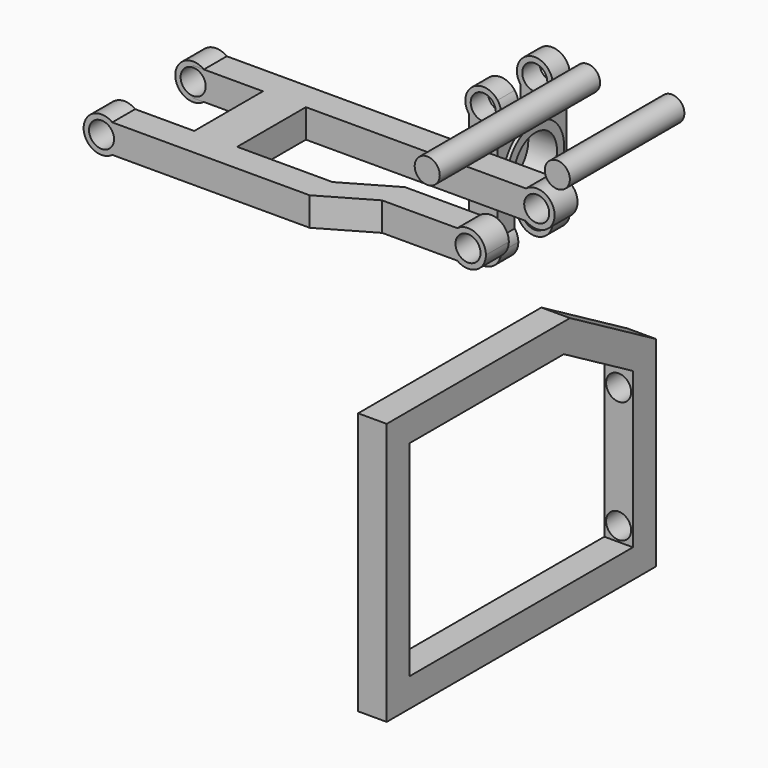
from build123d import *

# Parameters (mm, degrees)
F0_W      = 304.8
F0_H      = 25.4
F1_DEPTH  = 25.4
F4_DEPTH  = 25.4
F5_DEPTH  = 25.4
F7_DEPTH  = 25.4
F8_R      = 11.1125
F9_DEPTH  = 127.001
F10_R     = 11.1125
F11_DEPTH = 101.601
F12_R     = 11.1125
F13_DEPTH = 127.001
F14_W     = 38.1
F14_H     = 86.0915481232
F15_DEPTH = 25.4
F16_DEPTH = 25.4
F19_DEPTH = 12.7
F20_DEPTH = 12.7
F18_R     = 6.35
F21_DEPTH = 15.875
F23_DEPTH = 19.05
F24_DEPTH = 211.7314750923
F26_DEPTH = 19.05
F27_R     = 23.8125
F28_DEPTH = 25.4
F29_R     = 11.1125
F30_DEPTH = 127
F33_DEPTH = 25.4
F34_R     = 11.1125
F35_DEPTH = 25.4
F31_R     = 11.1125
F36_DEPTH = 177.8


# Not quite as in the source:
# - a pattern or mirror of a feature is missing from the dataset's text; its kind, count and spacing are read off the source's solid


with BuildPart() as f1:
    # F0 (on Top) → F1 (new body)
    with BuildSketch(Plane.XY):
        with Locations((-77.8089873464, -4.2339627839)):
            Rectangle(F0_W, F0_H)
    extrude(amount=F1_DEPTH)



with BuildPart() as f1b:
    # F0 (on Top) → F1, piece 2 (new body)
    with BuildSketch(Plane.XY):
        Polygon((-230.2089873464, -93.1339627839), (-230.2089873464, -118.5339627839), (-45.6030778587, -118.5339627839), (-1.6089873464, -93.1339627839), (74.5910126536, -93.1339627839), (74.5910126536, -67.7339627839), (-1.6089873464, -67.7339627839), (-45.6030778587, -93.1339627839), align=None)
    extrude(amount=F1_DEPTH)

    # F2 (on face) → F4 (join)
    with BuildSketch(Plane.XZ.offset(118.5339627839)):
        with BuildLine():
            Line((-230.2089873464, 25.4), (-220.6839873464, 25.4))
            ThreePointArc((-220.6839873464, 25.4), (-246.0839873464, 12.7), (-220.6839873464, 0))
            Line((-220.6839873464, 0), (-230.2089873464, 0))
            Line((-230.2089873464, 0), (-230.2089873464, 25.4))
        make_face()
    f4 = extrude(amount=-F4_DEPTH)

    # F4_copies: F4 across plane
    add(f4.mirror(Plane.ZX.offset(-55.033963)))

    # F3 (on face) → F5 (join)
    with BuildSketch(Plane.XZ.offset(93.1339627839)):
        with BuildLine():
            ThreePointArc((65.0660126536, 0), (81.6905284821, -1.4990316571), (90.4660126536, 12.7))
            ThreePointArc((90.4660126536, 12.7), (81.6905284821, 26.8990316571), (65.0660126536, 25.4))
            Line((65.0660126536, 25.4), (74.5910126536, 25.4))
            Line((74.5910126536, 25.4), (74.5910126536, 0))
            Line((74.5910126536, 0), (65.0660126536, 0))
        make_face()
        with BuildLine():
            Line((74.5910126536, 25.4), (65.0660126536, 25.4))
            ThreePointArc((65.0660126536, 25.4), (58.7160126536, 12.7), (65.0660126536, 0))
            Line((65.0660126536, 0), (74.5910126536, 0))
            Line((74.5910126536, 0), (74.5910126536, 25.4))
        make_face()
    extrude(amount=-F5_DEPTH)


with BuildPart() as f1_1:
    add(f1.part)

    add(f1b.part)  # F7 merges F1b
    # F6 (on face) → F7 (join)
    with BuildSketch(Plane(origin=(0, 8.4660372161, 0), x_dir=(-1, 0, 0), z_dir=(0, 1, 0))):
        with BuildLine():
            Line((-74.5910126536, 25.4), (-65.0660126536, 25.4))
            ThreePointArc((-65.0660126536, 25.4), (-90.4660126536, 12.7), (-65.0660126536, 0))
            Line((-65.0660126536, 0), (-74.5910126536, 0))
            Line((-74.5910126536, 0), (-74.5910126536, 25.4))
        make_face()
        with BuildLine():
            Line((230.2089873464, 25.4), (220.6839873464, 25.4))
            ThreePointArc((220.6839873464, 25.4), (214.3339873464, 12.7), (220.6839873464, 0))
            Line((220.6839873464, 0), (230.2089873464, 0))
            Line((230.2089873464, 0), (230.2089873464, 25.4))
        make_face()
    extrude(amount=-F7_DEPTH)

    # F8 (on face) → F9 (cut, through all)
    with BuildSketch(Plane.XZ.offset(118.5339627839)):
        with Locations((-230.2089873464, 12.7)):
            Circle(F8_R)
    extrude(amount=-F9_DEPTH, mode=Mode.SUBTRACT)

    # F10 (on face) → F11 (cut, through all)
    with BuildSketch(Plane.XZ.offset(93.1339627839)):
        with Locations((74.5910126536, 12.7)):
            Circle(F10_R)
    extrude(amount=-F11_DEPTH, mode=Mode.SUBTRACT)

    # F12 (on face) → F13 (cut, through all)
    with BuildSketch(Plane(origin=(0, 8.4660372161, 0), x_dir=(-1, 0, 0), z_dir=(0, 1, 0))):
        with Locations((-74.5910126536, 12.7)):
            Circle(F12_R)
        with BuildLine():
            ThreePointArc((230.2089873464, 1.5875), (238.0667114524, 4.8422758941), (241.3214873464, 12.7))
            ThreePointArc((241.3214873464, 12.7), (238.0667114524, 20.5577241059), (230.2089873464, 23.8125))
            ThreePointArc((230.2089873464, 23.8125), (222.3512632405, 20.5577241059), (219.0964873464, 12.7))
            ThreePointArc((219.0964873464, 12.7), (222.3512632405, 4.8422758941), (230.2089873464, 1.5875))
        make_face()
    extrude(amount=-F13_DEPTH, mode=Mode.SUBTRACT)

    # F14 (on face) → F15 (join)
    with BuildSketch(Plane.XY.offset(25.4)):
        with Locations((-149.2464873464, -59.9797368456)):
            Rectangle(F14_W, F14_H)
    extrude(amount=-F15_DEPTH)


with BuildPart() as f16:
    # F16 (new): a face of the model
    f16_faces = [f1_1.part.faces().sort_by_distance(p)[0] for p in [
        (-168.2964873464, -55.0339627839, 12.7),
    ]]
    extrude(f16_faces, amount=F16_DEPTH)


with BuildPart() as f19:
    # F18 (on Right) → F19 (new body, symmetric)
    with BuildSketch(Plane.YZ):
        with BuildLine():
            Line((36.0465123084, 63.5), (16.9965123084, 63.5))
            Line((16.9965123084, 63.5), (16.9965123084, -63.5))
            Line((16.9965123084, -63.5), (36.0465123084, -63.5))
            Line((36.0465123084, -63.5), (36.0465123084, -25.4))
            ThreePointArc((36.0465123084, -25.4), (23.3465123084, 0), (36.0465123084, 25.4))
            Line((36.0465123084, 25.4), (36.0465123084, 63.5))
        make_face()
    extrude(amount=F19_DEPTH, both=True)



with BuildPart() as f20:
    # F18 (on Right) → F20 (new body, symmetric)
    with BuildSketch(Plane.YZ):
        with BuildLine():
            Line((74.1465123084, 63.5), (74.1465123084, 25.4))
            ThreePointArc((74.1465123084, 25.4), (83.4945756227, 14.1990316571), (86.8465123084, 0))
            ThreePointArc((86.8465123084, 0), (83.4945756227, -14.1990316571), (74.1465123084, -25.4))
            Line((74.1465123084, -25.4), (74.1465123084, -63.5))
            Line((74.1465123084, -63.5), (93.1965123084, -63.5))
            Line((93.1965123084, -63.5), (93.1965123084, 63.5))
            Line((93.1965123084, 63.5), (74.1465123084, 63.5))
        make_face()
    extrude(amount=F20_DEPTH, both=True)


with BuildPart() as f19_1:
    add(f19.part)

    add(f20.part)  # F21 merges F20
    # F18 (on Right) → F21 (join, symmetric)
    with BuildSketch(Plane.YZ):
        with BuildLine():
            ThreePointArc((74.1465123084, 25.4), (55.0965123084, 31.75), (36.0465123084, 25.4))
            Line((36.0465123084, 25.4), (36.0465123084, 12.7))
            Line((36.0465123084, 12.7), (74.1465123084, 12.7))
            Line((74.1465123084, 12.7), (74.1465123084, 25.4))
        make_face()
        with BuildLine():
            Line((36.0465123084, 12.7), (36.0465123084, 25.4))
            ThreePointArc((36.0465123084, 25.4), (23.3465123084, 0), (36.0465123084, -25.4))
            Line((36.0465123084, -25.4), (36.0465123084, -12.7))
            Line((36.0465123084, -12.7), (74.1465123084, -12.7))
            Line((74.1465123084, -12.7), (74.1465123084, -25.4))
            ThreePointArc((74.1465123084, -25.4), (83.4945756227, -14.1990316571), (86.8465123084, 0))
            ThreePointArc((86.8465123084, 0), (83.4945756227, 14.1990316571), (74.1465123084, 25.4))
            Line((74.1465123084, 25.4), (74.1465123084, 12.7))
            Line((74.1465123084, 12.7), (36.0465123084, 12.7))
        make_face()
        with Locations((55.0965123084, 0)):
            Circle(F18_R, mode=Mode.SUBTRACT)
        with BuildLine():
            Line((36.0465123084, -12.7), (36.0465123084, -25.4))
            ThreePointArc((36.0465123084, -25.4), (55.0965123084, -31.75), (74.1465123084, -25.4))
            Line((74.1465123084, -25.4), (74.1465123084, -12.7))
            Line((74.1465123084, -12.7), (36.0465123084, -12.7))
        make_face()
        with BuildLine():
            ThreePointArc((74.1465123084, 25.4), (55.0965123084, 31.75), (36.0465123084, 25.4))
            Line((36.0465123084, 25.4), (36.0465123084, 12.7))
            Line((36.0465123084, 12.7), (74.1465123084, 12.7))
            Line((74.1465123084, 12.7), (74.1465123084, 25.4))
        make_face()
        with BuildLine():
            Line((36.0465123084, 12.7), (36.0465123084, 25.4))
            ThreePointArc((36.0465123084, 25.4), (23.3465123084, 0), (36.0465123084, -25.4))
            Line((36.0465123084, -25.4), (36.0465123084, -12.7))
            Line((36.0465123084, -12.7), (74.1465123084, -12.7))
            Line((74.1465123084, -12.7), (74.1465123084, -25.4))
            ThreePointArc((74.1465123084, -25.4), (83.4945756227, -14.1990316571), (86.8465123084, 0))
            ThreePointArc((86.8465123084, 0), (83.4945756227, 14.1990316571), (74.1465123084, 25.4))
            Line((74.1465123084, 25.4), (74.1465123084, 12.7))
            Line((74.1465123084, 12.7), (36.0465123084, 12.7))
        make_face()
        with Locations((55.0965123084, 0)):
            Circle(F18_R, mode=Mode.SUBTRACT)
        with BuildLine():
            Line((36.0465123084, -12.7), (36.0465123084, -25.4))
            ThreePointArc((36.0465123084, -25.4), (55.0965123084, -31.75), (74.1465123084, -25.4))
            Line((74.1465123084, -25.4), (74.1465123084, -12.7))
            Line((74.1465123084, -12.7), (36.0465123084, -12.7))
        make_face()
        with BuildLine():
            Line((36.0465123084, 12.7), (36.0465123084, 25.4))
            ThreePointArc((36.0465123084, 25.4), (23.3465123084, 0), (36.0465123084, -25.4))
            Line((36.0465123084, -25.4), (36.0465123084, -12.7))
            Line((36.0465123084, -12.7), (74.1465123084, -12.7))
            Line((74.1465123084, -12.7), (74.1465123084, -25.4))
            ThreePointArc((74.1465123084, -25.4), (83.4945756227, -14.1990316571), (86.8465123084, 0))
            ThreePointArc((86.8465123084, 0), (83.4945756227, 14.1990316571), (74.1465123084, 25.4))
            Line((74.1465123084, 25.4), (74.1465123084, 12.7))
            Line((74.1465123084, 12.7), (36.0465123084, 12.7))
        make_face()
        with Locations((55.0965123084, 0)):
            Circle(F18_R, mode=Mode.SUBTRACT)
    extrude(amount=F21_DEPTH, both=True)

    # F22 (on face) → F23 (join)
    with BuildSketch(Plane(origin=(0, 93.1965123084, 0), x_dir=(-1, 0, 0), z_dir=(0, 1, 0))):
        with BuildLine():
            Line((12.7, 44.45), (12.7, 63.5))
            Line((12.7, 63.5), (5.7238126498, 63.5))
            ThreePointArc((5.7238126498, 63.5), (9.6719575144, 59.4468273081), (11.1125, 53.975))
            ThreePointArc((11.1125, 53.975), (-5.4718273081, 44.3030424856), (-5.7238126498, 63.5))
            Line((-5.7238126498, 63.5), (-12.7, 63.5))
            Line((-12.7, 63.5), (-12.7, 44.45))
            ThreePointArc((-12.7, 44.45), (0, 38.1), (12.7, 44.45))
        make_face()
        with BuildLine():
            Line((-12.7, 44.45), (-12.7, 63.5))
            ThreePointArc((-12.7, 63.5), (-15.875, 53.975), (-12.7, 44.45))
        make_face()
        with BuildLine():
            ThreePointArc((12.7, 44.45), (15.0603473566, 48.9548842145), (15.875, 53.975))
            ThreePointArc((15.875, 53.975), (15.0603473566, 58.9951157855), (12.7, 63.5))
            Line((12.7, 63.5), (12.7, 44.45))
        make_face()
        with BuildLine():
            Line((5.7238126498, 63.5), (12.7, 63.5))
            ThreePointArc((12.7, 63.5), (0, 69.85), (-12.7, 63.5))
            Line((-12.7, 63.5), (-5.7238126498, 63.5))
            ThreePointArc((-5.7238126498, 63.5), (0, 65.0875), (5.7238126498, 63.5))
        make_face()
        with BuildLine():
            Line((-5.7238126498, 63.5), (5.7238126498, 63.5))
            ThreePointArc((5.7238126498, 63.5), (0, 65.0875), (-5.7238126498, 63.5))
        make_face()
        with BuildLine():
            ThreePointArc((15.875, -53.975), (15.0603473566, -48.9548842145), (12.7, -44.45))
            Line((12.7, -44.45), (12.7, -63.5))
            ThreePointArc((12.7, -63.5), (15.0603473566, -58.9951157855), (15.875, -53.975))
        make_face()
        with BuildLine():
            Line((12.7, -63.5), (12.7, -44.45))
            ThreePointArc((12.7, -44.45), (0, -38.1), (-12.7, -44.45))
            Line((-12.7, -44.45), (-12.7, -63.5))
            Line((-12.7, -63.5), (-5.7238126498, -63.5))
            ThreePointArc((-5.7238126498, -63.5), (-5.4718273081, -44.3030424856), (11.1125, -53.975))
            ThreePointArc((11.1125, -53.975), (9.6719575144, -59.4468273081), (5.7238126498, -63.5))
            Line((5.7238126498, -63.5), (12.7, -63.5))
        make_face()
        with BuildLine():
            ThreePointArc((-12.7, -63.5), (0, -69.85), (12.7, -63.5))
            Line((12.7, -63.5), (5.7238126498, -63.5))
            ThreePointArc((5.7238126498, -63.5), (0, -65.0875), (-5.7238126498, -63.5))
            Line((-5.7238126498, -63.5), (-12.7, -63.5))
        make_face()
        with BuildLine():
            Line((-12.7, -63.5), (-12.7, -44.45))
            ThreePointArc((-12.7, -44.45), (-15.875, -53.975), (-12.7, -63.5))
        make_face()
    extrude(amount=-F23_DEPTH)

    # F22 (on face) → F24 (cut, through all)
    with BuildSketch(Plane(origin=(0, 93.1965123084, 0), x_dir=(-1, 0, 0), z_dir=(0, 1, 0))):
        with BuildLine():
            ThreePointArc((11.1125, 53.975), (9.6719575144, 59.4468273081), (5.7238126498, 63.5))
            Line((5.7238126498, 63.5), (-5.7238126498, 63.5))
            ThreePointArc((-5.7238126498, 63.5), (-5.4718273081, 44.3030424856), (11.1125, 53.975))
        make_face()
        with BuildLine():
            Line((-5.7238126498, 63.5), (5.7238126498, 63.5))
            ThreePointArc((5.7238126498, 63.5), (0, 65.0875), (-5.7238126498, 63.5))
        make_face()
        with BuildLine():
            Line((-5.7238126498, -63.5), (5.7238126498, -63.5))
            ThreePointArc((5.7238126498, -63.5), (9.6719575144, -59.4468273081), (11.1125, -53.975))
            ThreePointArc((11.1125, -53.975), (-5.4718273081, -44.3030424856), (-5.7238126498, -63.5))
        make_face()
        with BuildLine():
            ThreePointArc((-5.7238126498, -63.5), (0, -65.0875), (5.7238126498, -63.5))
            Line((5.7238126498, -63.5), (-5.7238126498, -63.5))
        make_face()
    extrude(amount=-F24_DEPTH, mode=Mode.SUBTRACT)

    # F25 (on face) → F26 (join)
    with BuildSketch(Plane.XZ.offset(-16.9965123084)):
        with BuildLine():
            ThreePointArc((12.7, 44.45), (15.0603473566, 48.9548842145), (15.875, 53.975))
            ThreePointArc((15.875, 53.975), (15.0603473566, 58.9951157855), (12.7, 63.5))
            Line((12.7, 63.5), (12.7, 44.45))
        make_face()
        with BuildLine():
            Line((5.7238126498, 63.5), (12.7, 63.5))
            ThreePointArc((12.7, 63.5), (0, 69.85), (-12.7, 63.5))
            Line((-12.7, 63.5), (-5.7238126498, 63.5))
            ThreePointArc((-5.7238126498, 63.5), (0, 65.0875), (5.7238126498, 63.5))
        make_face()
        with BuildLine():
            Line((12.7, 44.45), (12.7, 63.5))
            Line((12.7, 63.5), (5.7238126498, 63.5))
            ThreePointArc((5.7238126498, 63.5), (9.6719575144, 59.4468273081), (11.1125, 53.975))
            ThreePointArc((11.1125, 53.975), (-5.4718273081, 44.3030424856), (-5.7238126498, 63.5))
            Line((-5.7238126498, 63.5), (-12.7, 63.5))
            Line((-12.7, 63.5), (-12.7, 44.45))
            ThreePointArc((-12.7, 44.45), (0, 38.1), (12.7, 44.45))
        make_face()
        with BuildLine():
            Line((-12.7, 44.45), (-12.7, 63.5))
            ThreePointArc((-12.7, 63.5), (-15.875, 53.975), (-12.7, 44.45))
        make_face()
        with BuildLine():
            Line((12.7, -63.5), (12.7, -44.45))
            ThreePointArc((12.7, -44.45), (0, -38.1), (-12.7, -44.45))
            Line((-12.7, -44.45), (-12.7, -63.5))
            Line((-12.7, -63.5), (-5.7238126498, -63.5))
            ThreePointArc((-5.7238126498, -63.5), (-5.4718273081, -44.3030424856), (11.1125, -53.975))
            ThreePointArc((11.1125, -53.975), (9.6719575144, -59.4468273081), (5.7238126498, -63.5))
            Line((5.7238126498, -63.5), (12.7, -63.5))
        make_face()
        with BuildLine():
            ThreePointArc((15.875, -53.975), (15.0603473566, -48.9548842145), (12.7, -44.45))
            Line((12.7, -44.45), (12.7, -63.5))
            ThreePointArc((12.7, -63.5), (15.0603473566, -58.9951157855), (15.875, -53.975))
        make_face()
        with BuildLine():
            Line((-12.7, -63.5), (-12.7, -44.45))
            ThreePointArc((-12.7, -44.45), (-15.875, -53.975), (-12.7, -63.5))
        make_face()
        with BuildLine():
            ThreePointArc((-12.7, -63.5), (0, -69.85), (12.7, -63.5))
            Line((12.7, -63.5), (5.7238126498, -63.5))
            ThreePointArc((5.7238126498, -63.5), (0, -65.0875), (-5.7238126498, -63.5))
            Line((-5.7238126498, -63.5), (-12.7, -63.5))
        make_face()
    extrude(amount=-F26_DEPTH)

    # F27 (on face) → F28 (cut)
    with BuildSketch(Plane.YZ.offset(15.875)):
        with Locations((55.0965123084, 0)):
            Circle(F27_R)
    extrude(amount=-F28_DEPTH, mode=Mode.SUBTRACT)


with BuildPart() as f30:
    # F29 (on Front) → F30 (new body)
    with BuildSketch(Plane.XZ):
        with Locations((180.9120774269, 118.5125783086)):
            Circle(F29_R)
    extrude(amount=F30_DEPTH)


with BuildPart() as f33:
    # F32 (on Right) → F33 (new body)
    with BuildSketch(Plane.YZ):
        Polygon((81.4398276971, -128.7355077243), (-121.7601723029, -128.7355077243), (-121.7601723029, -310.7051673555), (-121.7601723029, -361.5051673555), (176.6500710531, -361.5051673555), (176.6500710531, -183.7051673555), align=None)
        Polygon((-96.3601723029, -336.1051673555), (-96.3601723029, -154.1355077243), (74.6339182094, -154.1355077243), (151.2500710531, -198.3698641929), (151.2500710531, -336.1051673555), align=None, mode=Mode.SUBTRACT)
    extrude(amount=F33_DEPTH)

    # F34 (on face) → F35 (cut, through all)
    with BuildSketch(Plane(origin=(0, 176.6500710531, 0), x_dir=(-1, 0, 0), z_dir=(0, 1, 0))):
        with Locations((-12.7, -215.4551673555)):
            Circle(F34_R)
        with Locations((-12.7, -323.4051673555)):
            Circle(F34_R)
    extrude(amount=-F35_DEPTH, mode=Mode.SUBTRACT)


with BuildPart() as f36:
    # F31 (on Front) → F36 (new body)
    with BuildSketch(Plane.XZ):
        with Locations((106.1509624124, 118.070371449)):
            Circle(F31_R)
    extrude(amount=F36_DEPTH)


solid = Compound([f1_1.part, f19_1.part, f30.part, f33.part, f36.part])
